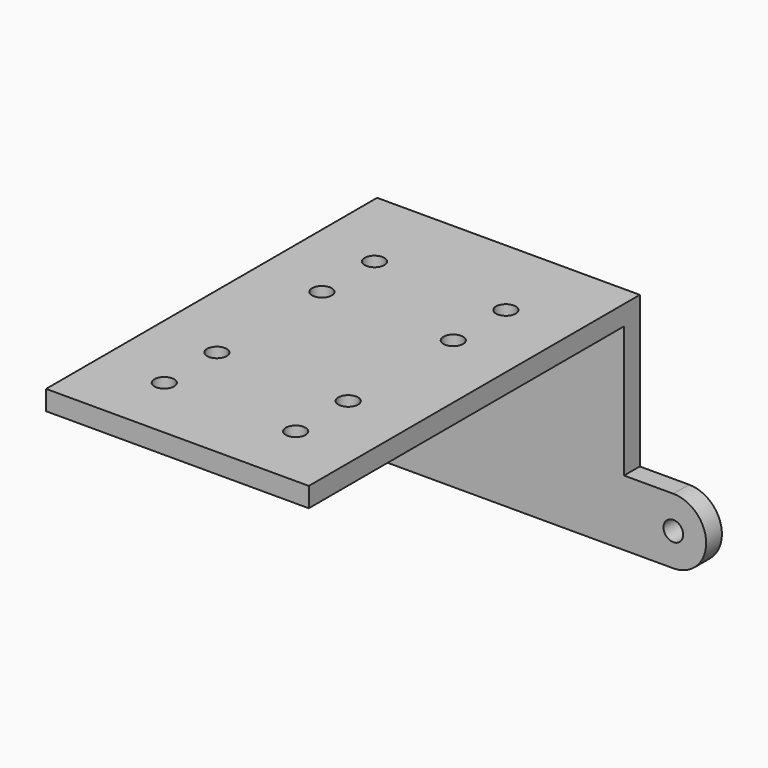
from build123d import *

# Parameters (mm, degrees)
F0_R     = 1.5
F1_DEPTH = 3
F2_R     = 1.5
F3_DEPTH = 3


# Not quite as in the source:
# - a feature names something its author has since deleted; it is built from what else it names


with BuildPart() as f1:
    # F0 (on Front) → F1 (new body)
    with BuildSketch(Plane.XZ):
        with BuildLine():
            Line((57.5, 5), (50, 5))
            Line((50, 5), (50, 25))
            Line((50, 25), (10, 25))
            Line((10, 25), (10, 5))
            Line((10, 5), (2.5, 5))
            ThreePointArc((2.5, 5), (-2.5, 0), (2.5, -5))
            Line((2.5, -5), (57.5, -5))
            ThreePointArc((57.5, -5), (62.5, 0), (57.5, 5))
        make_face()
        with Locations((2.5, 0)):
            Circle(F0_R, mode=Mode.SUBTRACT)
        with Locations((57.5, 0)):
            Circle(F0_R, mode=Mode.SUBTRACT)
    extrude(amount=F1_DEPTH)

    # F2 (on face) → F3 (join)
    with BuildSketch(Plane.XY.offset(25)):
        Polygon((50, 0), (10, 0), (10, -3), (10, -13), (10, -23), (10, -33), (10, -43), (10, -53), (10, -63), (50, -63), (50, -53), (50, -43), (50, -33), (50, -23), (50, -13), (50, -3), align=None)
        with BuildLine():
            ThreePointArc((21.5, -53), (20, -54.5), (18.5, -53))
            ThreePointArc((18.5, -53), (20, -51.5), (21.5, -53))
        make_face(mode=Mode.SUBTRACT)
        with BuildLine():
            ThreePointArc((21.5, -43), (20, -44.5), (18.5, -43))
            ThreePointArc((18.5, -43), (20, -41.5), (21.5, -43))
        make_face(mode=Mode.SUBTRACT)
        with Locations((40, -53)):
            Circle(F2_R, mode=Mode.SUBTRACT)
        with Locations((40, -43)):
            Circle(F2_R, mode=Mode.SUBTRACT)
        with BuildLine():
            ThreePointArc((21.5, -23), (20, -24.5), (18.5, -23))
            ThreePointArc((18.5, -23), (20, -21.5), (21.5, -23))
        make_face(mode=Mode.SUBTRACT)
        with BuildLine():
            ThreePointArc((21.5, -13), (20, -14.5), (18.5, -13))
            ThreePointArc((18.5, -13), (20, -11.5), (21.5, -13))
        make_face(mode=Mode.SUBTRACT)
        with Locations((40, -23)):
            Circle(F2_R, mode=Mode.SUBTRACT)
        with Locations((40, -13)):
            Circle(F2_R, mode=Mode.SUBTRACT)
    extrude(amount=F3_DEPTH)


solid = f1.part
